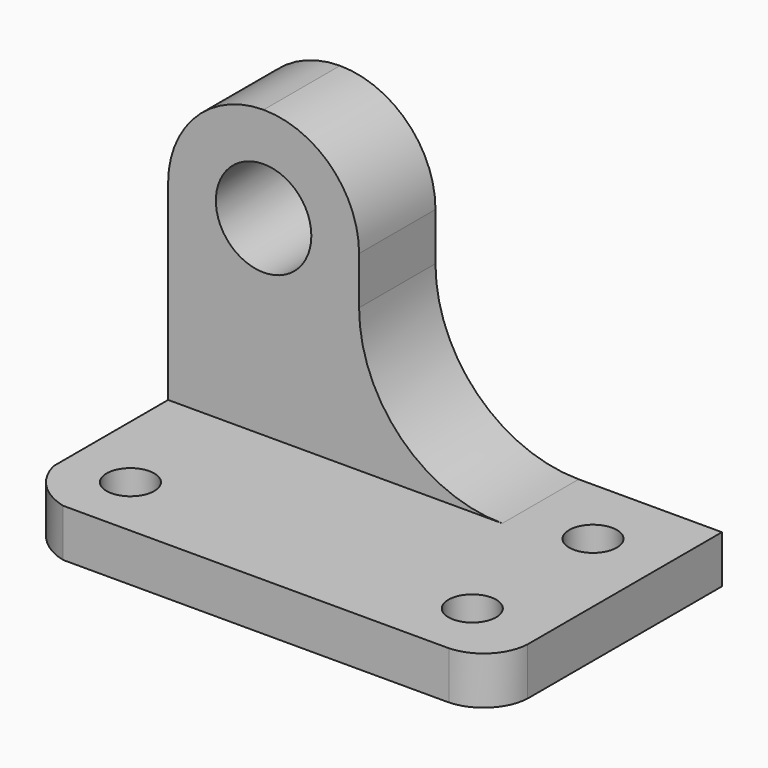
from build123d import *

# Parameters (mm, degrees)
F0_W      = 63.5
F0_H      = 38.1
F1_DEPTH  = 6.35
F2_W      = 44.45
F2_H      = 12.7
F3_DEPTH  = 38.1
F4_R      = 6.35
F5_DEPTH  = 25.4
F7_DEPTH  = 25.4
F10_DEPTH = 25.4
F12_DEPTH = 25.4
F13_R     = 3.175
F14_DEPTH = 25.4
F15_DEPTH = 25.4


# Not quite as in the source:
# - a feature names something its author has since deleted; it is built from what else it names


with BuildPart() as f1:
    # F0 (on Top) → F1 (new body)
    with BuildSketch(Plane.XY):
        with Locations((31.75, 19.05)):
            Rectangle(F0_W, F0_H)
    extrude(amount=F1_DEPTH)

    # F2 (on face) → F3 (join)
    with BuildSketch(Plane.XY.offset(6.35)):
        with Locations((22.225, 31.75)):
            Rectangle(F2_W, F2_H)
    extrude(amount=F3_DEPTH)

    # F4 (on face) → F5 (cut)
    with BuildSketch(Plane.XZ.offset(-25.4)):
        with Locations((12.7, 31.75)):
            Circle(F4_R)
    extrude(amount=-F5_DEPTH, mode=Mode.SUBTRACT)

    # F6 (on face) → F7 (cut)
    with BuildSketch(Plane.XZ.offset(-25.4)):
        with BuildLine():
            ThreePointArc((0, 31.7500000601), (3.7197439043, 40.7302561464), (12.7000000115, 44.45))
            Line((12.7000000115, 44.45), (0, 44.45))
            Line((0, 44.45), (0, 31.7500000601))
        make_face()
    extrude(amount=-F7_DEPTH, mode=Mode.SUBTRACT)

    # F9 (on face) → F10 (cut)
    with BuildSketch(Plane.XY.offset(6.35)):
        with BuildLine():
            ThreePointArc((6.35, 0), (2.3008253722, 2.3008253722), (0, 6.35))
            Line((0, 6.35), (0, 0))
            Line((0, 0), (6.35, 0))
        make_face()
    extrude(amount=-F10_DEPTH, mode=Mode.SUBTRACT)

    # F11 (on face) → F12 (cut)
    with BuildSketch(Plane.XY.offset(6.35)):
        with BuildLine():
            ThreePointArc((63.5, 5.8150525234), (61.7226257638, 1.7773742362), (57.6849474766, 0))
            Line((57.6849474766, 0), (63.5, 0))
            Line((63.5, 0), (63.5, 5.8150525234))
        make_face()
    extrude(amount=-F12_DEPTH, mode=Mode.SUBTRACT)

    # F13 (on face) → F14 (cut)
    with BuildSketch(Plane.XY.offset(6.35)):
        with Locations((53.975, 28.575)):
            Circle(F13_R)
        with Locations((53.975, 8.5037086033)):
            Circle(F13_R)
        with Locations((8.5037086033, 8.5037086033)):
            Circle(F13_R)
    extrude(amount=-F14_DEPTH, mode=Mode.SUBTRACT)

    # F8 (on face) → F15 (cut)
    with BuildSketch(Plane.XZ.offset(-25.4)):
        with BuildLine():
            ThreePointArc((12.7000000115, 44.45), (21.6802561251, 40.730256117), (25.4, 31.75))
            Line((25.4, 31.75), (25.4, 25.4))
            ThreePointArc((25.4, 25.4), (30.9796158184, 11.9296158184), (44.45, 6.35))
            Line((44.45, 6.35), (44.45, 44.45))
            Line((44.45, 44.45), (12.7000000115, 44.45))
        make_face()
    extrude(amount=-F15_DEPTH, mode=Mode.SUBTRACT)


solid = f1.part
